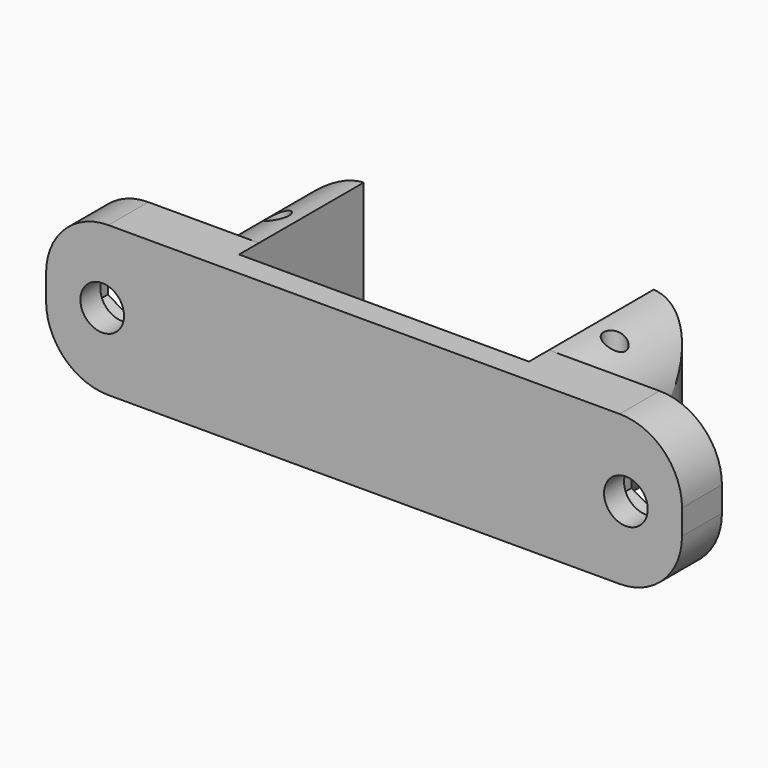
from build123d import *

# Parameters (mm, degrees)
F0_R        = 0.875
F1_DEPTH    = 12
F2_R        = 1.75
F3_DEPTH    = 25
F4_DEPTH    = 2
F5_T1_DEPTH = 36.9921862789
F5_T3_DEPTH = 29
F5_T5_DEPTH = 22.9960931395


# Not quite as in the source:
# - a fillet or chamfer that OpenCascade refuses, or shapes differently, is made with other operations: its cross-section is extruded or revolved along the edge and cut away or added


with BuildPart() as f1:
    # F0 (on Top) → F1 (new body)
    with BuildSketch(Plane.XY):
        Polygon((-11.625, 7.25), (-16.5, 7.25), (-16.5, -3.25), (-16.5, -5.25), (-11.625, -5.25), align=None)
        with Locations((-13.5, 1)):
            Circle(F0_R, mode=Mode.SUBTRACT)
        Polygon((-16.5, -5.25), (-16.5, -3.25), (-25.5, -3.25), (-25.5, -7.25), (-16.5, -7.25), align=None)
        Polygon((11.625, -5.25), (-11.625, -5.25), (-16.5, -5.25), (-16.5, -7.25), (16.5, -7.25), (16.5, -5.25), align=None)
        Polygon((25.5, -3.25), (16.5, -3.25), (16.5, -5.25), (16.5, -7.25), (25.5, -7.25), align=None)
        Polygon((16.5, 7.25), (11.625, 7.25), (11.625, -5.25), (16.5, -5.25), (16.5, -3.25), align=None)
        with Locations((13.5, 1)):
            Circle(F0_R, mode=Mode.SUBTRACT)
    extrude(amount=F1_DEPTH)

    # F2 (on face) → F3 (cut)
    with BuildSketch(Plane(origin=(0, -3.25, 0), x_dir=(-1, 0, 0), z_dir=(0, 1, 0))):
        with Locations((-21, 6)):
            Circle(F2_R)
        with Locations((21, 6)):
            Circle(F2_R)
    extrude(amount=-F3_DEPTH, mode=Mode.SUBTRACT)

    # F2 (on face) → F4 (cut)
    with BuildSketch(Plane(origin=(0, -3.25, 0), x_dir=(-1, 0, 0), z_dir=(0, 1, 0))):
        Polygon((-23.75, 7.5877132403), (-23.75, 4.4122867597), (-21, 2.8245735195), (-18.25, 4.4122867597), (-18.25, 7.5877132403), (-21, 9.1754264805), align=None)
        with Locations((-21, 6)):
            Circle(F2_R, mode=Mode.SUBTRACT)
        Polygon((23.75, 4.4122867597), (23.75, 7.5877132403), (21, 9.1754264805), (18.25, 7.5877132403), (18.25, 4.4122867597), (21, 2.8245735195), align=None)
        with Locations((21, 6)):
            Circle(F2_R, mode=Mode.SUBTRACT)
    extrude(amount=-F4_DEPTH, mode=Mode.SUBTRACT)

    # F5: fillet of radius 5 on 10 edges, made by hand

    # F5_s2 → F5_t1 (cut)
    with BuildSketch(Plane.XY.offset(-12.4960931395)):
        with BuildLine():
            ThreePointArc((-11.625, 7.25), (-15.0794552658, 5.7426227552), (-16.5, 2.2515627442))
            Line((-16.5, 2.2515627442), (-16.5, 7.25))
            Line((-16.5, 7.25), (-11.625, 7.25))
        make_face()
        with BuildLine():
            ThreePointArc((16.5, 2.2515627442), (15.0794552658, 5.7426227552), (11.625, 7.25))
            Line((11.625, 7.25), (16.5, 7.25))
            Line((16.5, 7.25), (16.5, 2.2515627442))
        make_face()
    extrude(amount=F5_T1_DEPTH, mode=Mode.SUBTRACT)

    # F5_s4 → F5_t3 (cut)
    with BuildSketch(Plane.XZ.offset(-9.25)):
        with BuildLine():
            ThreePointArc((20.5, 12), (24.0355339059, 10.5355339059), (25.5, 7))
            Line((25.5, 7), (25.5, 12))
            Line((25.5, 12), (20.5, 12))
        make_face()
        with BuildLine():
            ThreePointArc((20.5, 0), (24.0355339059, 1.4644660941), (25.5, 5))
            Line((25.5, 5), (25.5, 0))
            Line((25.5, 0), (20.5, 0))
        make_face()
        with BuildLine():
            ThreePointArc((-20.5, 0), (-24.0355339059, 1.4644660941), (-25.5, 5))
            Line((-25.5, 5), (-25.5, 0))
            Line((-25.5, 0), (-20.5, 0))
        make_face()
        with BuildLine():
            ThreePointArc((-20.5, 12), (-24.0355339059, 10.5355339059), (-25.5, 7))
            Line((-25.5, 7), (-25.5, 12))
            Line((-25.5, 12), (-20.5, 12))
        make_face()
    extrude(amount=F5_T3_DEPTH, mode=Mode.SUBTRACT)

    # F5_s6 → F5_t5 (cut)
    with BuildSketch(Plane.XZ.offset(-19.7460931395)):
        with BuildLine():
            ThreePointArc((11.625, 0), (15.0794552658, 1.5073772448), (16.5, 4.9984372558))
            Line((16.5, 4.9984372558), (16.5, 0))
            Line((16.5, 0), (11.625, 0))
        make_face()
        with BuildLine():
            ThreePointArc((11.625, 12), (15.0794552658, 10.4926227552), (16.5, 7.0015627442))
            Line((16.5, 7.0015627442), (16.5, 12))
            Line((16.5, 12), (11.625, 12))
        make_face()
        with BuildLine():
            ThreePointArc((-16.5, 7.0015627442), (-15.0794552658, 10.4926227552), (-11.625, 12))
            Line((-11.625, 12), (-16.5, 12))
            Line((-16.5, 12), (-16.5, 7.0015627442))
        make_face()
        with BuildLine():
            ThreePointArc((-16.5, 4.9984372558), (-15.0794552658, 1.5073772448), (-11.625, 0))
            Line((-11.625, 0), (-16.5, 0))
            Line((-16.5, 0), (-16.5, 4.9984372558))
        make_face()
    extrude(amount=F5_T5_DEPTH, mode=Mode.SUBTRACT)


solid = f1.part
